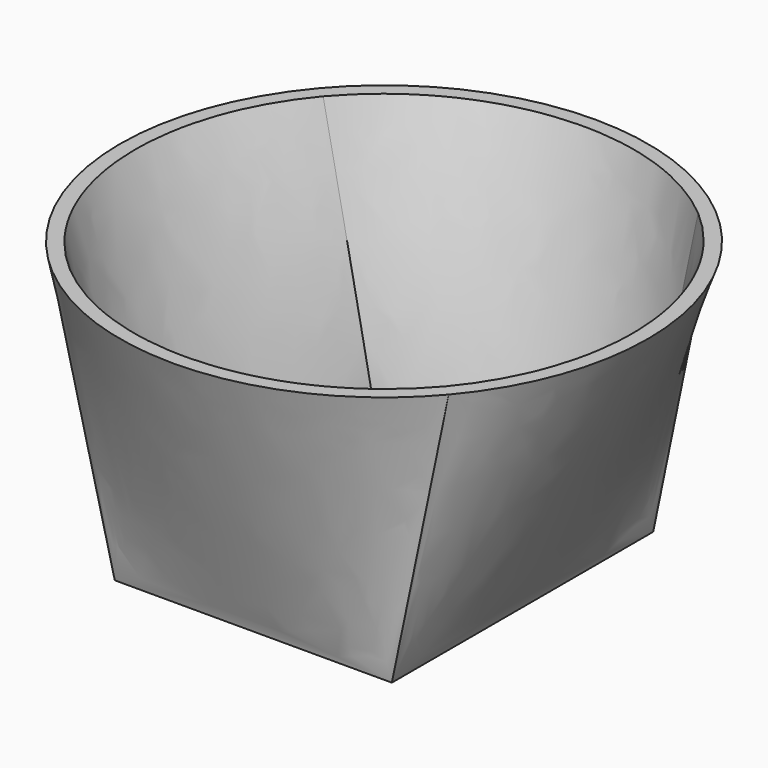
from build123d import *

# Parameters (mm, degrees)
F0_W = 50.8
F0_H = 59.9056573934
F4_T = 2.54


# Not quite as in the source:
# - the arcs of a loft's sections are written as splines that run evenly, so that the points pair up as in the source's solid
# - a shell that OpenCascade refuses in one call is made with other operations: the cavity is built on its own and cut out


with BuildPart() as f3:
    # F2 (on offset) → F3 section 0
    with BuildSketch(Plane.XY.offset(50.8)):
        with BuildLine():
            add(Edge.make_bspline(
                [(31.3033898449, 36.9143729784), (28.8873497832, 38.9631750527), (26.269585061, 40.7739731742), (20.7309490894, 43.8501509409), (17.8102147937, 45.1154545216), (11.7778696482, 47.0519901199), (8.66640796, 47.7231742528), (2.3721732815, 48.4456477056), (-0.8104440715, 48.4969191609), (-7.1246843741, 47.9775662186), (-10.2561511918, 47.406954663), (-16.3477444048, 45.6657337679), (-19.3077201735, 44.4951674836), (-24.9425697859, 41.5989927782), (-27.6173042968, 39.8734559709), (-32.5788661981, 35.9336258251), (-34.865570904, 33.7194299066), (-36.9143729784, 31.3033898449)],
                knots=[0, 0, 0, 0, 0.125, 0.125, 0.25, 0.25, 0.375, 0.375, 0.5, 0.5, 0.625, 0.625, 0.75, 0.75, 0.875, 0.875, 1, 1, 1, 1], degree=3))
            add(Edge.make_bspline(
                [(-36.9143729784, 31.3033898449), (-38.9631750527, 28.8873497832), (-40.7739731742, 26.269585061), (-43.8501509409, 20.7309490894), (-45.1154545216, 17.8102147937), (-47.0519901199, 11.7778696482), (-47.7231742528, 8.66640796), (-48.4456477056, 2.3721732815), (-48.4969191609, -0.8104440715), (-47.9775662186, -7.1246843741), (-47.406954663, -10.2561511918), (-45.6657337679, -16.3477444048), (-44.4951674836, -19.3077201735), (-41.5989927782, -24.9425697859), (-39.8734559709, -27.6173042968), (-35.9336258251, -32.5788661981), (-33.7194299066, -34.865570904), (-31.3033898449, -36.9143729784)],
                knots=[0, 0, 0, 0, 0.125, 0.125, 0.25, 0.25, 0.375, 0.375, 0.5, 0.5, 0.625, 0.625, 0.75, 0.75, 0.875, 0.875, 1, 1, 1, 1], degree=3))
            add(Edge.make_bspline(
                [(-31.3033898449, -36.9143729784), (-28.8873497832, -38.9631750527), (-26.269585061, -40.7739731742), (-20.7309490894, -43.8501509409), (-17.8102147937, -45.1154545216), (-11.7778696482, -47.0519901199), (-8.66640796, -47.7231742528), (-2.3721732815, -48.4456477056), (0.8104440715, -48.4969191609), (7.1246843741, -47.9775662186), (10.2561511918, -47.406954663), (16.3477444048, -45.6657337679), (19.3077201735, -44.4951674836), (24.9425697859, -41.5989927782), (27.6173042968, -39.8734559709), (32.5788661981, -35.9336258251), (34.865570904, -33.7194299066), (36.9143729784, -31.3033898449)],
                knots=[0, 0, 0, 0, 0.125, 0.125, 0.25, 0.25, 0.375, 0.375, 0.5, 0.5, 0.625, 0.625, 0.75, 0.75, 0.875, 0.875, 1, 1, 1, 1], degree=3))
            add(Edge.make_bspline(
                [(36.9143729784, -31.3033898449), (38.9631750527, -28.8873497832), (40.7739731742, -26.269585061), (43.8501509409, -20.7309490894), (45.1154545216, -17.8102147937), (47.0519901199, -11.7778696482), (47.7231742528, -8.66640796), (48.4456477056, -2.3721732815), (48.4969191609, 0.8104440715), (47.9775662186, 7.1246843741), (47.406954663, 10.2561511918), (45.6657337679, 16.3477444048), (44.4951674836, 19.3077201735), (41.5989927782, 24.9425697859), (39.8734559709, 27.6173042968), (35.9336258251, 32.5788661981), (33.7194299066, 34.865570904), (31.3033898449, 36.9143729784)],
                knots=[0, 0, 0, 0, 0.125, 0.125, 0.25, 0.25, 0.375, 0.375, 0.5, 0.5, 0.625, 0.625, 0.75, 0.75, 0.875, 0.875, 1, 1, 1, 1], degree=3))
        make_face()
    # F0 (on Top) → F3 section 1
    with BuildSketch(Plane.XY):
        Rectangle(F0_W, F0_H)
    loft(ruled=True)

    # F4: shell of thickness 2.54, made by hand


with BuildPart() as f4_core1:
    # F4_t2: copy of F3
    add(f3.part)

    # the walls: a layer under each face that stays
    f4_faces = [f4_core1.faces().sort_by_distance(p)[0] for p in [
        (-1.9837821114, 39.0950356932, 25.4),
        (-36.8186213449, -1.9837821114, 25.4),
        (1.9837821114, -39.0950356932, 25.4),
        (36.8186213449, 1.9837821114, 25.4),
        (0, 0, 0),
    ]]
    thicken(f4_faces, amount=-F4_T, mode=Mode.SUBTRACT)


with BuildPart() as f3_1:
    add(f3.part)

    # what is left inside the walls is the cavity
    f4_cavity = [f4_core1.part.solids().sort_by_distance(p)[0] for p in [
        (11.647477, -9.877061, 50.7746),
    ]]
    add(f4_cavity, mode=Mode.SUBTRACT)


solid = f3_1.part
